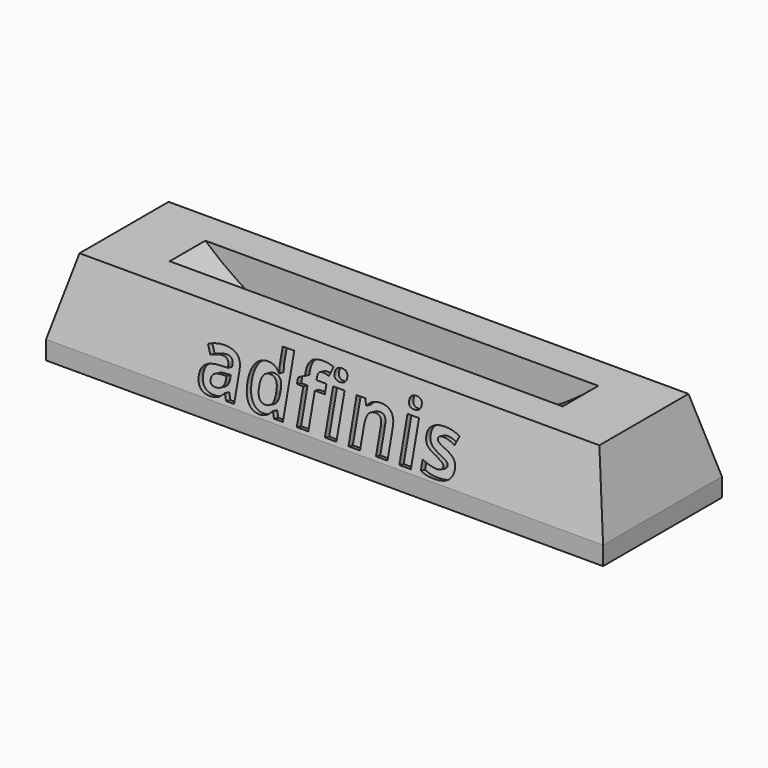
from build123d import *

# Parameters (mm, degrees)
F0_W         = 30
F0_H         = 4
F1_DEPTH     = 5
F2_SIZE2     = 4
F2_SIZE      = 1
F4_DEPTH     = 1.2
F6_TEXT_SIZE = 4.1666666667
F7_DEPTH     = 0.3
F8_TEXT_SIZE = 4.1666666667
F9_DEPTH     = 0.3


# Not quite as in the source:
# - Text() gives the source's letters only with a copy of the font that has no kerning and outlines rounded to 1/6400 em; it was checked with that copy


with BuildPart() as f1:
    # F0 (on Top) → F1 (new body)
    with BuildSketch(Plane.XY):
        Rectangle(F0_W, F0_H)
    extrude(amount=F1_DEPTH)

    # F2
    f2_edges = [f1.edges().sort_by_distance(p)[0] for p in [
        (0, 2, 5),
        (-15, 0, 5),
        (15, 0, 5),
    ]]
    f2_side = f1.faces().sort_by_distance((0, 0, 5))[0]
    chamfer(f2_edges, length=F2_SIZE, length2=F2_SIZE2, reference=f2_side)

    # F3 (on face) → F4 (cut)
    with BuildSketch(Plane.XZ.offset(2)):
        with BuildLine():
            Line((10.5830052443, 5), (-10.5830052443, 5))
            ThreePointArc((-10.5830052443, 5), (0, 1), (10.5830052443, 5))
        make_face()
    extrude(amount=-F4_DEPTH, mode=Mode.SUBTRACT)

    # F5: F1 across face


with BuildPart() as f1_1:
    add(f1.part)
    add(f1.part.mirror(Plane(origin=(0, -2, 1.8655599645), x_dir=(1, 0, 0), z_dir=(0, -1, 0))))

    # F6 (on face) → F7 (cut)
    with BuildSketch(Plane(origin=(0, 2.1176470588, 0.5294117647), x_dir=(-1, 0, 0), z_dir=(0, 0.9701425001, 0.242535625))):
        with Locations((-7.1155598958, 0.6850712501)):
            Text('adfinis', F6_TEXT_SIZE, font='Open Sans', font_style=FontStyle.BOLD, text_align=(TextAlign.LEFT, TextAlign.BOTTOM))
    extrude(amount=-F7_DEPTH, mode=Mode.SUBTRACT)

    # F8 (on face) → F9 (cut)
    with BuildSketch(Plane(origin=(0, -5.8823529412, 1.4705882353), x_dir=(1, 0, 0), z_dir=(0, -0.9701425001, 0.242535625))):
        with Locations((-7.1155598958, -0.2850712501)):
            Text('adfinis', F8_TEXT_SIZE, font='Open Sans', font_style=FontStyle.BOLD, text_align=(TextAlign.LEFT, TextAlign.BOTTOM))
    extrude(amount=-F9_DEPTH, mode=Mode.SUBTRACT)


solid = f1_1.part
